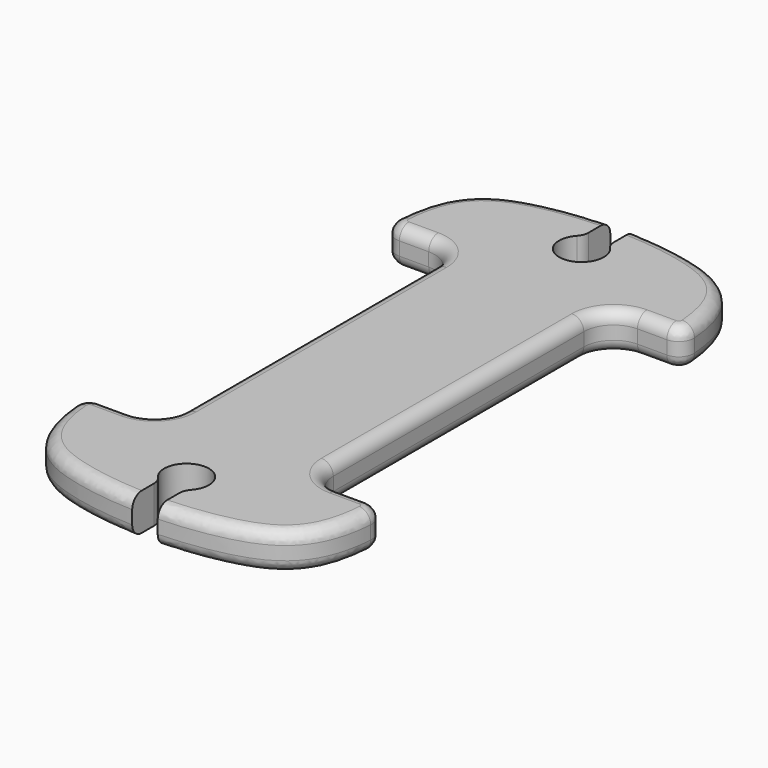
from build123d import *

# Parameters (mm, degrees)
F1_DEPTH = 2.5
F2_R     = 2
F3_R     = 1
F4_R     = 0.8
F6_DEPTH = 2.5010001
F7_R     = 1


# Not quite as in the source:
# - a pattern or mirror of a feature is missing from the dataset's text; its kind, count and spacing are read off the source's solid


with BuildPart() as f1:
    # F0 (on Top) → F1 (new body)
    with BuildSketch(Plane.XY):
        with BuildLine():
            Line((-10, 12.5), (-5, 12.5))
            Line((-5, 12.5), (-5, -12.5))
            Line((-5, -12.5), (-10, -12.5))
            add(Edge.make_bspline(
                [(-10, -12.5), (-10, -17.5), (-5.5198760922, -20.2365921043), (5.5198760922, -20.2365921043), (10, -17.5), (10, -12.5)],
                knots=[0, 0, 0, 0, 0.3248670825, 0.6751329175, 1, 1, 1, 1], degree=3))
            Line((10, -12.5), (5, -12.5))
            Line((5, -12.5), (5, 12.5))
            Line((5, 12.5), (10, 12.5))
            add(Edge.make_bspline(
                [(-10, 12.5), (-10, 17.5), (-5.5198760922, 20.2365921043), (5.5198760922, 20.2365921043), (10, 17.5), (10, 12.5)],
                knots=[0, 0, 0, 0, 0.3248670825, 0.6751329175, 1, 1, 1, 1], degree=3))
        make_face()
    extrude(amount=F1_DEPTH)

    # F2
    f2_edges = [f1.edges().sort_by_distance(p)[0] for p in [
        (-5, 12.5, 1.25),
        (5, 12.5, 1.25),
        (5, -12.5, 1.25),
        (-5, -12.5, 1.25),
    ]]
    fillet(f2_edges, radius=F2_R)

    # F3
    f3_edges = [f1.edges().sort_by_distance(p)[0] for p in [
        (-10, -12.5, 1.25),
        (10, -12.5, 1.25),
        (10, 12.5, 1.25),
        (-10, 12.5, 1.25),
    ]]
    fillet(f3_edges, radius=F3_R)

    # F4
    f4_edges = [f1.edges().sort_by_distance(p)[0] for p in [
        (-7.983139, 12.5, 2.5),
        (-9.698029, 12.818429, 2.5),
        (-5.585786, 11.914214, 2.5),
        (0, 20.052444, 2.5),
        (-5, 0, 2.5),
        (9.698029, 12.818429, 2.5),
        (-5.585786, -11.914214, 2.5),
        (7.983139, 12.5, 2.5),
        (-7.983139, -12.5, 2.5),
        (5.585786, 11.914214, 2.5),
        (-9.698029, -12.818429, 2.5),
        (5, 0, 2.5),
        (0, -20.052444, 2.5),
        (5.585786, -11.914214, 2.5),
        (9.698029, -12.818429, 2.5),
        (7.983139, -12.5, 2.5),
        (-7.983139, 12.5, 0),
        (-9.698029, 12.818429, 0),
        (-5.585786, 11.914214, 0),
        (0, 20.052444, 0),
        (-5, 0, 0),
        (9.698029, 12.818429, 0),
        (-5.585786, -11.914214, 0),
        (7.983139, 12.5, 0),
        (-7.983139, -12.5, 0),
        (5.585786, 11.914214, 0),
        (-9.698029, -12.818429, 0),
        (5, 0, 0),
        (0, -20.052444, 0),
        (5.585786, -11.914214, 0),
        (9.698029, -12.818429, 0),
        (7.983139, -12.5, 0),
    ]]
    fillet(f4_edges, radius=F4_R)

    # F5 (on face) → F6 (cut, through all)
    with BuildSketch(Plane.XY.offset(2.5)):
        with BuildLine():
            ThreePointArc((0.8556297795, -17.7844739806), (1.3291810767, -17.2476258281), (1.5, -16.5524440782))
            ThreePointArc((1.5, -16.5524440782), (-0.6951817499, -15.2232630015), (-0.8556297795, -17.7844739806))
            Line((-0.8556297795, -17.7844739806), (0.8556297795, -17.7844739806))
        make_face()
        with BuildLine():
            Line((0.8556297795, -17.7844739806), (-0.8556297795, -17.7844739806))
            ThreePointArc((-0.8556297795, -17.7844739806), (0, -18.0524440782), (0.8556297795, -17.7844739806))
        make_face()
        with BuildLine():
            ThreePointArc((0.8556297795, -17.7844739806), (0, -18.0524440782), (-0.8556297795, -17.7844739806))
            Line((-0.8556297795, -17.7844739806), (-0.8556297795, -24.4006932874))
            Line((-0.8556297795, -24.4006932874), (0.8556297795, -24.4006932874))
            Line((0.8556297795, -24.4006932874), (0.8556297795, -17.7844739806))
        make_face()
    f6 = extrude(amount=-F6_DEPTH, mode=Mode.SUBTRACT)

    # F6_copies: F6 across plane
    add(f6.mirror(Plane.ZX), mode=Mode.SUBTRACT)

    # F7
    f7_edges = [f1.edges().sort_by_distance(p)[0] for p in [
        (-0.85563, -17.784474, 1.25),
        (0.85563, -17.784474, 1.25),
        (-0.85563, 17.784474, 1.25),
        (0.85563, 17.784474, 1.25),
    ]]
    fillet(f7_edges, radius=F7_R)


solid = f1.part
